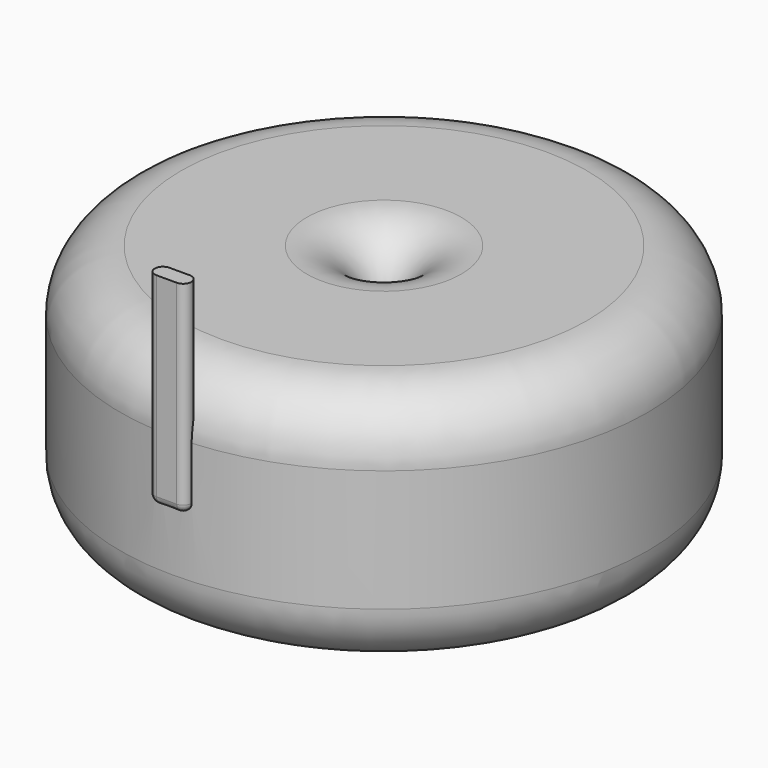
from build123d import *

# Parameters (mm, degrees)
F0_R     = 65
F0_R_2   = 4
F1_DEPTH = 30
F2_R     = 15
F4_DEPTH = 50
F5_R     = 1.9999


# Not quite as in the source:
# - a fillet or chamfer is up to 0.001 mm smaller than in the source, because OpenCascade refuses the exact size


with BuildPart() as f1:
    # F0 (on Top) → F1 (new body, symmetric)
    with BuildSketch(Plane.XY):
        Circle(F0_R)
        Circle(F0_R_2, mode=Mode.SUBTRACT)
    extrude(amount=F1_DEPTH, both=True)

    # F2
    f2_edges = [f1.edges().sort_by_distance(p)[0] for p in [
        (-4, 0, 30),
        (4, 0, 0),
        (-4, 0, -30),
        (-65, 0, -30),
        (65, 0, 0),
        (-65, 0, 30),
    ]]
    fillet(f2_edges, radius=F2_R)

    # F3 (on Top) → F4 (join)
    with BuildSketch(Plane.XY):
        with BuildLine():
            Line((2.5, -62.9519052838), (-2.5, -62.9519052838))
            ThreePointArc((-2.5, -62.9519052838), (-4.5, -64.9519052838), (-2.5, -66.9519052838))
            Line((-2.5, -66.9519052838), (2.5, -66.9519052838))
            ThreePointArc((2.5, -66.9519052838), (4.5, -64.9519052838), (2.5, -62.9519052838))
        make_face()
    extrude(amount=F4_DEPTH)

    # F5 (radius 2 in the source; OpenCascade refuses exactly that, so slightly less here)
    f5_edges = [f1.edges().sort_by_distance(p)[0] for p in [
        (0, -66.951905, 0),
    ]]
    fillet(f5_edges, radius=F5_R)


solid = f1.part
